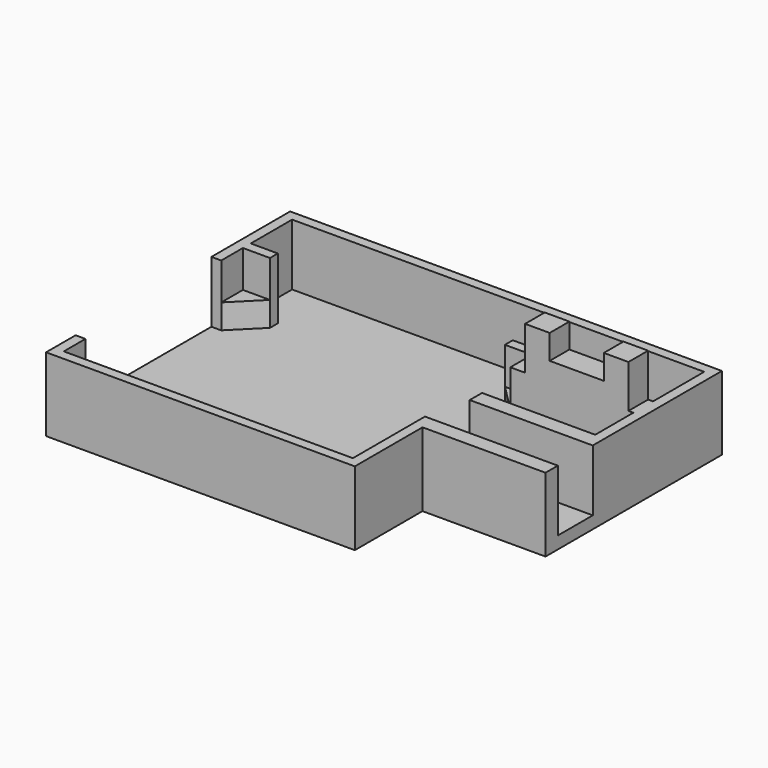
from build123d import *

# Parameters (mm, degrees)
F0_W     = 19.1
F0_H     = 0.8
F0_W_2   = 0.8
F0_H_2   = 13.8
F0_W_3   = 2.45
F0_H_3   = 1
F0_H_4   = 2
F0_W_4   = 4.3
F0_H_5   = 3.875
F0_W_5   = 9.2
F0_H_6   = 3.55
F0_H_7   = 1.25
F1_DEPTH = 1
F2_DEPTH = 2
F3_DEPTH = 5
F4_W     = 2
F4_H     = 2
F4_W_2   = 4.4
F5_DEPTH = 1.5
F6_W     = 2
F6_H     = 2
F7_DEPTH = 2


# Not quite as in the source:
# - a feature names something its author has since deleted; it is built from what else it names


with BuildPart() as f1:
    # F0 (on Top) → F1 (new body)
    with BuildSketch(Plane.XY):
        Polygon((-1.9181339439, 9.1929600332), (-1.1181339439, 9.1929600332), (-1.1181339439, 11.3929600332), (1.0818660561, 11.3929600332), (1.0818660561, 12.1929600332), (-1.1181339439, 12.1929600332), (-1.9181339439, 12.1929600332), align=None)
        Polygon((-1.1181339439, 11.3929600332), (-1.1181339439, 9.1929600332), (1.0818660561, 11.3929600332), align=None)
        with Locations((10.6318660561, 11.7929600332)):
            Rectangle(F0_W, F0_H)
        Polygon((1.0818660561, -6.8070399668), (20.1818660561, -6.8070399668), (22.3818660561, -4.6070399668), (22.3818660561, 0.5179600332), (22.3818660561, 9.1929600332), (20.1818660561, 11.3929600332), (1.0818660561, 11.3929600332), (-1.1181339439, 9.1929600332), (-1.1181339439, -4.6070399668), align=None)
        with Locations((-1.5181339439, 2.2929600332)):
            Rectangle(F0_W_2, F0_H_2)
        Polygon((-1.9181339439, -7.6070399668), (1.0818660561, -7.6070399668), (1.0818660561, -6.8070399668), (-1.1181339439, -6.8070399668), (-1.1181339439, -4.6070399668), (-1.9181339439, -4.6070399668), (-1.9181339439, -6.8070399668), align=None)
        Polygon((-1.1181339439, -6.8070399668), (1.0818660561, -6.8070399668), (-1.1181339439, -4.6070399668), align=None)
        with Locations((10.6318660561, -7.2070399668)):
            Rectangle(F0_W, F0_H)
        Polygon((20.1818660561, -7.6070399668), (23.1818660561, -7.6070399668), (23.1818660561, -4.6070399668), (22.3818660561, -4.6070399668), (22.3818660561, -6.8070399668), (20.1818660561, -6.8070399668), align=None)
        Polygon((22.3818660561, -4.6070399668), (20.1818660561, -6.8070399668), (22.3818660561, -6.8070399668), align=None)
        Polygon((22.3818660561, 0.5179600332), (23.1818660561, 0.5179600332), (23.1818660561, 4.0679600332), (23.1818660561, 5.3179600332), (23.1818660561, 9.1929600332), (22.3818660561, 9.1929600332), align=None)
        Polygon((20.1818660561, 11.3929600332), (22.3818660561, 9.1929600332), (22.3818660561, 11.3929600332), align=None)
        Polygon((22.3818660561, 11.3929600332), (22.3818660561, 9.1929600332), (23.1818660561, 9.1929600332), (23.1818660561, 11.1929600332), (23.1818660561, 12.1929600332), (20.1818660561, 12.1929600332), (20.1818660561, 11.3929600332), align=None)
        with Locations((24.4068660561, 11.6929600332)):
            Rectangle(F0_W_3, F0_H_3)
        with Locations((24.4068660561, 10.1929600332)):
            Rectangle(F0_W_3, F0_H_4)
        with Locations((27.7818660561, 10.1929600332)):
            Rectangle(F0_W_4, F0_H_4)
        with Locations((27.7818660561, 11.6929600332)):
            Rectangle(F0_W_4, F0_H_3)
        with Locations((31.1568660561, 7.2554600332)):
            Rectangle(F0_W_3, F0_H_5)
        Polygon((32.3818660561, 9.1929600332), (32.3818660561, 5.3179600332), (33.1818660561, 5.3179600332), (33.1818660561, 12.1929600332), (32.3818660561, 12.1929600332), (32.3818660561, 11.1929600332), align=None)
        with Locations((27.7818660561, 7.2554600332)):
            Rectangle(F0_W_4, F0_H_5)
        with Locations((24.4068660561, 7.2554600332)):
            Rectangle(F0_W_3, F0_H_5)
        Polygon((23.1818660561, 5.3179600332), (23.1818660561, 4.0679600332), (32.3818660561, 4.0679600332), (32.3818660561, 5.3179600332), (29.9318660561, 5.3179600332), (25.6318660561, 5.3179600332), align=None)
        with Locations((27.7818660561, 2.2929600332)):
            Rectangle(F0_W_5, F0_H_6)
        with Locations((27.7818660561, -0.1070399668)):
            Rectangle(F0_W_5, F0_H_7)
        with Locations((32.7818660561, -0.1070399668)):
            Rectangle(F0_W_2, F0_H_7)
        with Locations((32.7818660561, 2.2929600332)):
            Rectangle(F0_W_2, F0_H_6)
        with Locations((32.7818660561, 4.6929600332)):
            Rectangle(F0_W_2, F0_H_7)
        Polygon((-1.9181339439, 17.1929600332), (-1.9181339439, 12.1929600332), (-1.1181339439, 12.1929600332), (-1.1181339439, 16.3929600332), (23.1818660561, 16.3929600332), (25.6318660561, 16.3929600332), (29.9318660561, 16.3929600332), (32.3818660561, 16.3929600332), (32.3818660561, 12.1929600332), (33.1818660561, 12.1929600332), (33.1818660561, 17.1929600332), (29.9318660561, 17.1929600332), (25.6318660561, 17.1929600332), (23.1818660561, 17.1929600332), align=None)
        Polygon((1.0818660561, 12.1929600332), (20.1818660561, 12.1929600332), (23.1818660561, 12.1929600332), (25.6318660561, 12.1929600332), (29.9318660561, 12.1929600332), (32.3818660561, 12.1929600332), (32.3818660561, 16.3929600332), (29.9318660561, 16.3929600332), (25.6318660561, 16.3929600332), (23.1818660561, 16.3929600332), (-1.1181339439, 16.3929600332), (-1.1181339439, 12.1929600332), align=None)
        Polygon((22.3818660561, -4.6070399668), (23.1818660561, -4.6070399668), (23.1818660561, -0.7320399668), (23.1818660561, 0.5179600332), (22.3818660561, 0.5179600332), align=None)
        with Locations((31.1568660561, 10.1929600332)):
            Rectangle(F0_W_3, F0_H_4)
        with Locations((31.1568660561, 11.6929600332)):
            Rectangle(F0_W_3, F0_H_3)
    extrude(amount=-F1_DEPTH)

    # F0 (on Top) → F2 (join)
    with BuildSketch(Plane.XY):
        Polygon((-1.1181339439, -6.8070399668), (1.0818660561, -6.8070399668), (-1.1181339439, -4.6070399668), align=None)
        Polygon((22.3818660561, -4.6070399668), (20.1818660561, -6.8070399668), (22.3818660561, -6.8070399668), align=None)
        Polygon((20.1818660561, 11.3929600332), (22.3818660561, 9.1929600332), (22.3818660561, 11.3929600332), align=None)
        Polygon((-1.1181339439, 11.3929600332), (-1.1181339439, 9.1929600332), (1.0818660561, 11.3929600332), align=None)
    extrude(amount=F2_DEPTH)

    # F0 (on Top) → F3 (join)
    with BuildSketch(Plane.XY):
        Polygon((-1.9181339439, -7.6070399668), (1.0818660561, -7.6070399668), (1.0818660561, -6.8070399668), (-1.1181339439, -6.8070399668), (-1.1181339439, -4.6070399668), (-1.9181339439, -4.6070399668), (-1.9181339439, -6.8070399668), align=None)
        Polygon((-1.9181339439, 9.1929600332), (-1.1181339439, 9.1929600332), (-1.1181339439, 11.3929600332), (1.0818660561, 11.3929600332), (1.0818660561, 12.1929600332), (-1.1181339439, 12.1929600332), (-1.9181339439, 12.1929600332), align=None)
        Polygon((20.1818660561, -7.6070399668), (23.1818660561, -7.6070399668), (23.1818660561, -4.6070399668), (22.3818660561, -4.6070399668), (22.3818660561, -6.8070399668), (20.1818660561, -6.8070399668), align=None)
        Polygon((22.3818660561, 11.3929600332), (22.3818660561, 9.1929600332), (23.1818660561, 9.1929600332), (23.1818660561, 11.1929600332), (23.1818660561, 12.1929600332), (20.1818660561, 12.1929600332), (20.1818660561, 11.3929600332), align=None)
        Polygon((-1.9181339439, 17.1929600332), (-1.9181339439, 12.1929600332), (-1.1181339439, 12.1929600332), (-1.1181339439, 16.3929600332), (23.1818660561, 16.3929600332), (25.6318660561, 16.3929600332), (29.9318660561, 16.3929600332), (32.3818660561, 16.3929600332), (32.3818660561, 12.1929600332), (33.1818660561, 12.1929600332), (33.1818660561, 17.1929600332), (29.9318660561, 17.1929600332), (25.6318660561, 17.1929600332), (23.1818660561, 17.1929600332), align=None)
        Polygon((32.3818660561, 9.1929600332), (32.3818660561, 5.3179600332), (33.1818660561, 5.3179600332), (33.1818660561, 12.1929600332), (32.3818660561, 12.1929600332), (32.3818660561, 11.1929600332), align=None)
        with Locations((32.7818660561, 4.6929600332)):
            Rectangle(F0_W_2, F0_H_7)
        with Locations((32.7818660561, -0.1070399668)):
            Rectangle(F0_W_2, F0_H_7)
        with Locations((27.7818660561, -0.1070399668)):
            Rectangle(F0_W_5, F0_H_7)
        Polygon((22.3818660561, -4.6070399668), (23.1818660561, -4.6070399668), (23.1818660561, -0.7320399668), (23.1818660561, 0.5179600332), (22.3818660561, 0.5179600332), align=None)
        with Locations((27.7818660561, 10.1929600332)):
            Rectangle(F0_W_4, F0_H_4)
        with Locations((24.4068660561, 10.1929600332)):
            Rectangle(F0_W_3, F0_H_4)
        with Locations((31.1568660561, 10.1929600332)):
            Rectangle(F0_W_3, F0_H_4)
        Polygon((23.1818660561, 5.3179600332), (23.1818660561, 4.0679600332), (32.3818660561, 4.0679600332), (32.3818660561, 5.3179600332), (29.9318660561, 5.3179600332), (25.6318660561, 5.3179600332), align=None)
        with Locations((10.6318660561, -7.2070399668)):
            Rectangle(F0_W, F0_H)
    extrude(amount=F3_DEPTH)

    # F4 (on face) → F5 (join)
    with BuildSketch(Plane.XY.offset(5)):
        with Locations((30.9818660561, 10.1929600332)):
            Rectangle(F4_W, F4_H)
        with Locations((24.5818660561, 10.1929600332)):
            Rectangle(F4_W, F4_H)
        with Locations((27.7818660561, 10.1929600332)):
            Rectangle(F4_W_2, F4_H)
    extrude(amount=F5_DEPTH)

    # F6 (on face) → F7 (join)
    with BuildSketch(Plane.XY.offset(6.5)):
        with Locations((24.5818660561, 10.1929600332)):
            Rectangle(F6_W, F6_H)
        with Locations((30.9818660561, 10.1929600332)):
            Rectangle(F6_W, F6_H)
    extrude(amount=F7_DEPTH)


solid = f1.part
